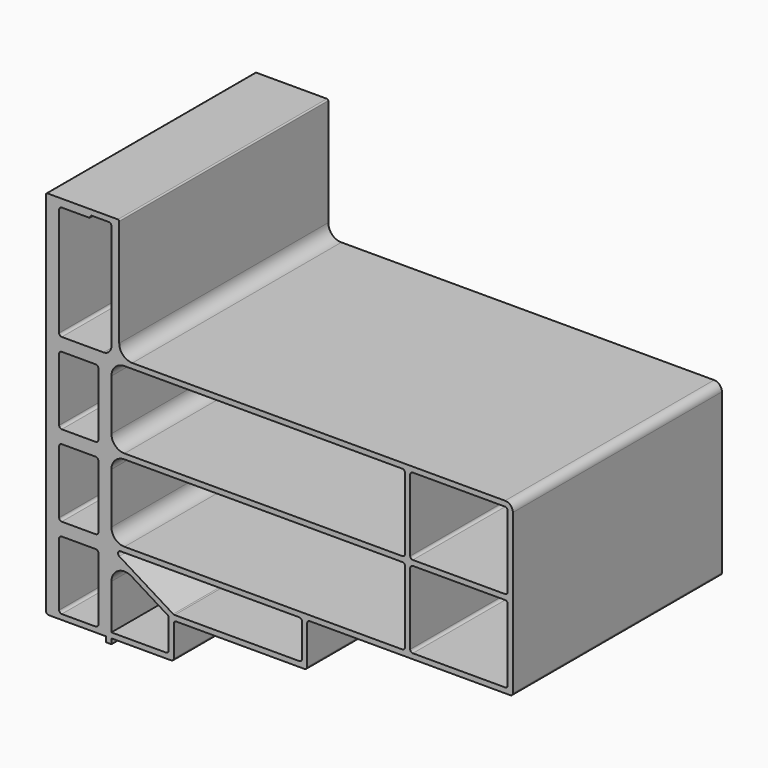
from build123d import *

# Parameters (mm, degrees)
F0_W     = 15
F0_H     = 26.12
F0_W_2   = 112.35
F0_H_2   = 29.4448914682
F0_W_3   = 37.3
F1_DEPTH = 100
F2_R     = 5
F3_R     = 1
F4_R     = 0.49999
F5_R     = 3


# Not quite as in the source:
# - two fillets or chamfers of one size are made in one step
# - a fillet or chamfer is up to 0.001 mm smaller than in the source, because OpenCascade refuses the exact size
# - a feature names something its author has since deleted; it is built from what else it names


with BuildPart() as f1:
    # F0 (on Front) → F1 (new body)
    with BuildSketch(Plane.XZ):
        Polygon((0, 141.95), (0, 0), (23, 0), (23, -2), (25, -2), (25, 0), (48.9, 0), (48.9, 13.7202170637), (99.9, 13.7202170637), (99.9, 30.4702170637), (178.65, 30.4702170637), (178.65, 95.36), (28, 95.36), (28, 141.95), align=None)
        with Locations((12.5, 15.06)):
            Rectangle(F0_W, F0_H, mode=Mode.SUBTRACT)
        Polygon((25, 2), (25, 28.12), (46.9, 14.6043096234), (46.9, 2), align=None, mode=Mode.SUBTRACT)
        Polygon((97.9, 15.7202170637), (48.9, 15.7202170637), (25, 30.4702170637), (97.9, 30.4702170637), align=None, mode=Mode.SUBTRACT)
        with Locations((12.5, 46.18)):
            Rectangle(F0_W, F0_H, mode=Mode.SUBTRACT)
        with Locations((81.175, 47.1926627978)):
            Rectangle(F0_W_2, F0_H_2, mode=Mode.SUBTRACT)
        with Locations((158, 47.1926627978)):
            Rectangle(F0_W_3, F0_H_2, mode=Mode.SUBTRACT)
        with Locations((12.5, 77.3)):
            Rectangle(F0_W, F0_H, mode=Mode.SUBTRACT)
        with Locations((81.175, 78.6375542659)):
            Rectangle(F0_W_2, F0_H_2, mode=Mode.SUBTRACT)
        Polygon((25, 95.36), (5, 95.36), (5, 138.95), (17, 138.95), (17, 139.95), (25, 139.95), align=None, mode=Mode.SUBTRACT)
        with Locations((158, 78.6375542659)):
            Rectangle(F0_W_3, F0_H_2, mode=Mode.SUBTRACT)
    extrude(amount=F1_DEPTH)

    # F2
    f2_edges = [f1.edges().sort_by_distance(p)[0] for p in [
        (28, -50, 95.36),
        (25, -50, 28.12),
        (25, -50, 32.470217),
        (25, -50, 61.915109),
        (25, -50, 93.36),
        (25, -50, 63.915109),
    ]]
    fillet(f2_edges, radius=F2_R)

    # F3
    f3_edges = [f1.edges().sort_by_distance(p)[0] for p in [
        (5, -50, 64.24),
        (5, -50, 33.12),
        (5, -50, 2),
        (5, -50, 90.36),
        (5, -50, 59.24),
        (5, -50, 28.12),
        (20, -50, 28.12),
        (20, -50, 59.24),
        (20, -50, 90.36),
        (20, -50, 64.24),
        (20, -50, 33.12),
        (20, -50, 2),
        (46.9, -50, 2),
        (46.9, -50, 14.60431),
        (25, -50, 30.470217),
        (97.9, -50, 15.720217),
        (97.9, -50, 30.470217),
        (137.35, -50, 61.915109),
        (137.35, -50, 93.36),
        (137.35, -50, 63.915109),
        (137.35, -50, 32.470217),
        (176.65, -50, 32.470217),
        (176.65, -50, 63.915109),
        (139.35, -50, 63.915109),
        (139.35, -50, 61.915109),
        (139.35, -50, 93.36),
        (176.65, -50, 93.36),
        (176.65, -50, 61.915109),
        (139.35, -50, 32.470217),
        (99.9, -50, 30.470217),
        (48.9, -50, 13.720217),
        (48.9, -50, 0),
        (0, -50, 0),
        (48.9, -50, 15.720217),
        (99.9, -50, 13.720217),
        (178.65, -50, 30.470217),
        (25, -50, 139.95),
        (5, -50, 95.36),
        (5, -50, 138.95),
    ]]
    fillet(f3_edges, radius=F3_R)

    # F4 (radius 0.5 in the source; OpenCascade refuses exactly that, so slightly less here)
    f4_edges = [f1.edges().sort_by_distance(p)[0] for p in [
        (0, -50, 141.95),
        (28, -50, 141.95),
        (17, -50, 139.95),
        (17, -50, 138.95),
    ]]
    fillet(f4_edges, radius=F4_R)

    # F5
    f5_edges = [f1.edges().sort_by_distance(p)[0] for p in [
        (178.65, -50, 95.36),
        (25, -50, 95.36),
    ]]
    fillet(f5_edges, radius=F5_R)


solid = f1.part
